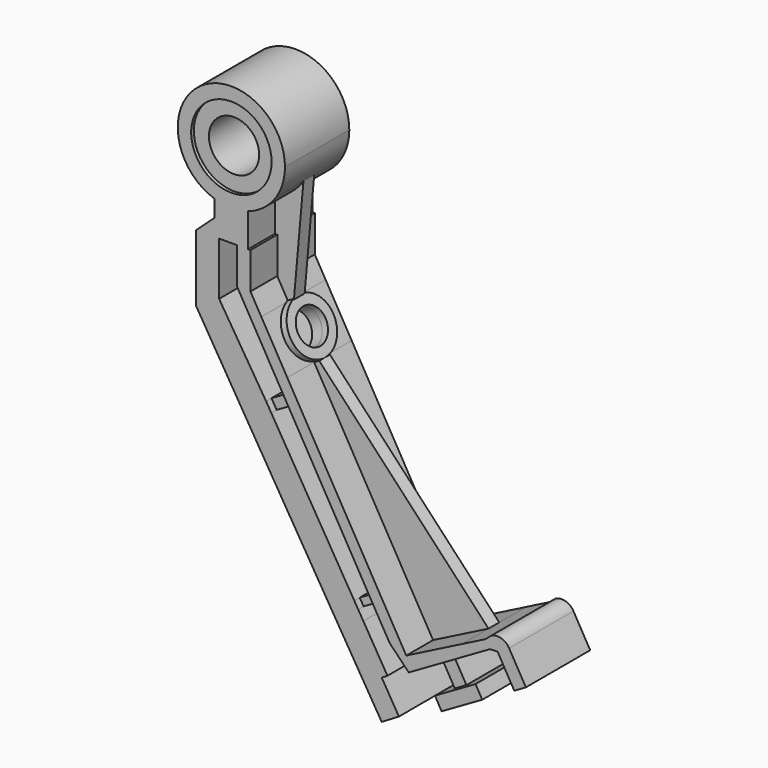
from build123d import *

# Parameters (mm, degrees)
F0_R     = 6
F1_DEPTH = 6
F2_DEPTH = 5
F0_R_2   = 3.75
F3_DEPTH = 5.5
F4_DEPTH = 1
F5_R     = 2.55
F6_DEPTH = 1
F7_DEPTH = 3


# Not quite as in the source:
# - a feature names something its author has since deleted; it is built from what else it names


with BuildPart() as f1:
    # F0 (on Front) → F1 (new body, symmetric)
    with BuildSketch(Plane.XZ):
        with BuildLine():
            ThreePointArc((6.7603327111, -4.2776046609), (7.6838356857, -2.2268069417), (8, 0))
            ThreePointArc((8, 0), (-4.6904157598, 6.4807406984), (-2.5, -7.5993420768))
            ThreePointArc((-2.5, -7.5993420768), (0, -8), (2.5, -7.5993420768))
            ThreePointArc((2.5, -7.5993420768), (4.9190370343, -6.3089677963), (6.7603327111, -4.2776046609))
        make_face()
        Circle(F0_R, mode=Mode.SUBTRACT)
        with BuildLine():
            ThreePointArc((2.5, -7.5993420768), (0, -8), (-2.5, -7.5993420768))
            Line((-2.5, -7.5993420768), (-2.5, -10.0993420768))
            Line((-2.5, -10.0993420768), (-2.5, -12.5993420768))
            Line((-2.5, -12.5993420768), (-1.8303241628, -12.5993420768))
            Line((-1.8303241628, -12.5993420768), (-1.25, -12.5993420768))
            Line((-1.25, -12.5993420768), (0, -12.5993420768))
            Line((0, -12.5993420768), (0.85, -12.5993420768))
            Line((0.85, -12.5993420768), (2.5, -12.5993420768))
            Line((2.5, -12.5993420768), (2.5, -7.5993420768))
        make_face()
        Polygon((-2.5, -12.5993420768), (-2.5, -10.0993420768), (-5.25, -12.5993420768), align=None)
        Polygon((2.85, -12.5993420768), (2.5, -12.5993420768), (0.85, -12.5993420768), (0.85, -18.0378015974), (2.85, -18.0378015974), align=None)
        Polygon((8.3499999998, -27.5640810386), (4.4667434126, -20.8380833309), (2.85, -18.0378015974), (0.85, -18.0378015974), (7.8499425387, -30.1621904255), (8.5998597667, -31.4610993824), (20.6315315697, -52.3007943349), (21.192894901, -53.2731147882), (21.8498235115, -54.4109609722), (23.5998091461, -57.4420581792), (25.0328148241, -58.9241157783), (26.1, -58.3079828733), align=None)
        with BuildLine():
            ThreePointArc((41.4522628248, -52.3492529341), (40.2378545238, -51.4173955261), (38.7202154867, -51.6171891785))
            Line((38.7202154867, -51.6171891785), (39.720207278, -53.3492447254))
            Line((39.720207278, -53.3492447254), (41.4522628248, -52.3492529341))
        make_face()
        Polygon((41.4522628248, -52.3492529341), (39.720207278, -53.3492447254), (42.2201867561, -57.6793835925), (43.9522423029, -56.6793918013), align=None)
        Polygon((-1.8303241628, -12.5993420768), (-2.5, -12.5993420768), (-5.25, -12.5993420768), (-5.25, -22.5993420768), (-1.8303241628, -20.5242957716), align=None)
        Polygon((-1.8303241628, -20.5242957716), (-5.25, -22.5993420768), (22.4316151512, -68.2186375255), (25.0052518507, -66.6770817727), (22.4359922626, -62.3876872736), (23.2938711624, -61.8738353559), (19.6969077391, -55.8686830572), (18.9284228965, -54.5804940001), (18.3501014099, -53.6179642353), (5.9549663233, -32.9881126107), (5.1864814807, -31.6999235536), align=None)
        Polygon((34.376104393, -54.107172761), (26.1, -58.3079828733), (25.0328148241, -58.9241157783), (26.4658205021, -60.4061733773), (30.7959593692, -57.9061938992), (32.5280149161, -56.906202108), (38.5902093302, -53.4062308387), (39.720207278, -53.3492447254), (38.7202154867, -51.6171891785), (37.9429287948, -52.2967132374), align=None)
    extrude(amount=F1_DEPTH, both=True)



with BuildPart() as f1b:
    # F0 (on Front) → F1, piece 2 (new body, symmetric)
    with BuildSketch(Plane.XZ):
        Polygon((34.2780005508, -59.937299315), (32.5459450039, -60.9372911063), (30.3808755703, -62.1872808453), (31.3808673616, -63.9193363922), (37.4430617756, -60.4193651228), (36.4430699844, -58.687309576), align=None)
    extrude(amount=F1_DEPTH, both=True)


with BuildPart() as f1_1:
    add(f1.part)

    add(f1b.part)  # F2 merges F1b
    # F0 (on Front) → F2 (join, symmetric)
    with BuildSketch(Plane.XZ):
        Polygon((32.5280149161, -56.906202108), (30.7959593692, -57.9061938992), (32.5459450039, -60.9372911063), (34.2780005508, -59.937299315), align=None)
        Polygon((8.5998597667, -31.4610993824), (7.8499425387, -30.1621904255), (5.1864814807, -31.6999235536), (5.9549663233, -32.9881126107), align=None)
        Polygon((21.192894901, -53.2731147882), (20.6315315697, -52.3007943349), (18.3501014099, -53.6179642353), (18.9284228965, -54.5804940001), align=None)
    extrude(amount=F2_DEPTH, both=True)

    # F0 (on Front) → F3 (join, symmetric)
    with BuildSketch(Plane.XZ):
        Circle(F0_R)
        Circle(F0_R_2, mode=Mode.SUBTRACT)
    extrude(amount=F3_DEPTH, both=True)

    # F0 (on Front) → F4 (join, symmetric)
    with BuildSketch(Plane.XZ):
        with BuildLine():
            Line((5.3327688164, -20.3380833309), (6.7603327111, -4.2776046609))
            ThreePointArc((6.7603327111, -4.2776046609), (4.9190370343, -6.3089677963), (2.5, -7.5993420768))
            Line((2.5, -7.5993420768), (2.5, -12.5993420768))
            Line((2.5, -12.5993420768), (2.85, -12.5993420768))
            Line((2.85, -12.5993420768), (2.85, -18.0378015974))
            Line((2.85, -18.0378015974), (4.4667434126, -20.8380833309))
            Line((4.4667434126, -20.8380833309), (5.3327688164, -20.3380833309))
        make_face()
        Polygon((9.1110238739, -27.1409636232), (8.3499999998, -27.5640810386), (26.1, -58.3079828733), (34.376104393, -54.107172761), align=None)
    extrude(amount=F4_DEPTH, both=True)

    # F5 (on face) → F6 (join)
    with BuildSketch(Plane(origin=(-5.6730972059, 0, -3.2753641989), x_dir=(0, 1, 0), z_dir=(0.8660254038, 0, 0.5))):
        with BuildLine():
            ThreePointArc((0, -28.0461944113), (2.8284271247, -26.8746215361), (4, -24.0461944113))
            ThreePointArc((4, -24.0461944113), (3.1622776602, -21.5967046686), (1, -20.1732110651))
            Line((1, -20.1732110651), (1, -20.279681237))
            Line((1, -20.279681237), (-1, -20.279681237))
            Line((-1, -20.279681237), (-1, -20.1732110651))
            ThreePointArc((-1, -20.1732110651), (-3.9681187851, -24.5502115813), (0, -28.0461944113))
        make_face()
        with Locations((0, -24.0461944113)):
            Circle(F5_R, mode=Mode.SUBTRACT)
    extrude(amount=F6_DEPTH)

    # F5 (on face) → F7 (cut)
    with BuildSketch(Plane(origin=(-5.6730972059, 0, -3.2753641989), x_dir=(0, 1, 0), z_dir=(0.8660254038, 0, 0.5))):
        with Locations((0, -24.0461944113)):
            Circle(F5_R)
    extrude(amount=-F7_DEPTH, mode=Mode.SUBTRACT)


solid = f1_1.part
